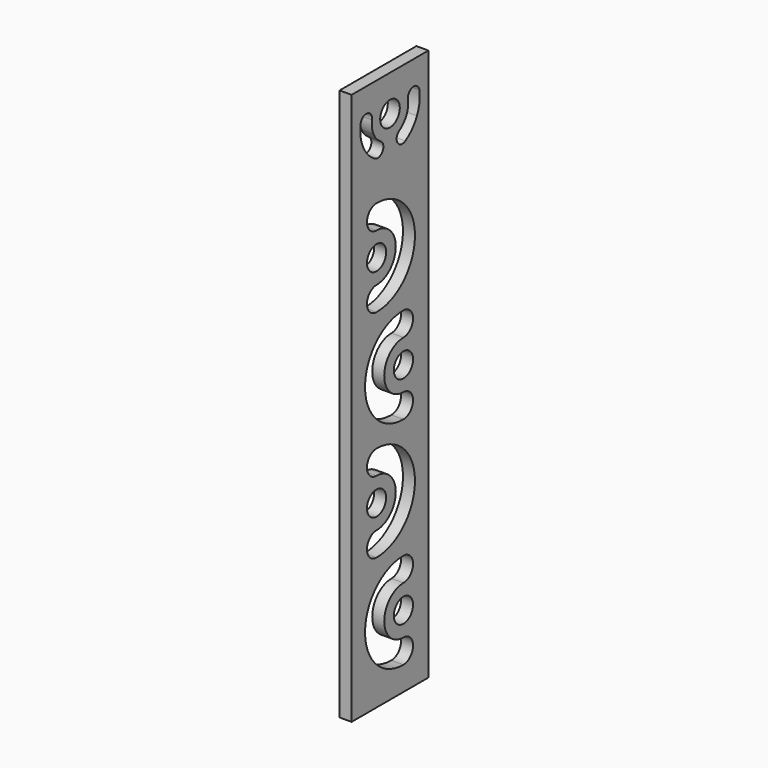
from build123d import *

# Parameters (mm, degrees)
F0_W      = 63.5
F0_H      = 63.5
F0_W_2    = 50.8
F0_H_2    = 50.8
F1_DEPTH  = 165.1
F3_R      = 6.477
F4_DEPTH  = 25.4
F6_DEPTH  = 25.4
F7_R      = 6.35
F8_DEPTH  = 63.501
F9_W      = 93.0855199695
F9_H      = 380.0157606602
F9_W_2    = 50.8
F9_H_2    = 292.1
F10_DEPTH = 38.1
F11_W     = 93.9574092627
F11_H     = 381.9095790386
F12_DEPTH = 91.44


# Not quite as in the source:
# - ends of sketch curves that miss each other by under 0.0002 mm in the source are joined


with BuildPart() as f1:
    # F0 (on Top) → F1 (new body, symmetric)
    with BuildSketch(Plane.XY):
        Rectangle(F0_W, F0_H)
        Rectangle(F0_W_2, F0_H_2, mode=Mode.SUBTRACT)
    extrude(amount=F1_DEPTH, both=True)

    # F3 (on face) → F4 (cut)
    with BuildSketch(Plane.YZ.offset(31.75)):
        with Locations((0, 146.05)):
            Circle(F3_R)
        with BuildLine():
            ThreePointArc((10.1385245046, 129.1766616857), (14.6288058895, 132.8781640138), (17.8406687878, 137.7307595176))
            ThreePointArc((17.8406687878, 137.7307595176), (19.4934269332, 143.3103775076), (19.4426449846, 149.1294124443))
            ThreePointArc((19.4426449846, 149.1294124443), (15.0835370951, 152.2964897102), (11.9164598293, 147.9373818207))
            ThreePointArc((11.9164598293, 147.9373818207), (11.9475842494, 144.3708765369), (10.9346034506, 140.9511106721))
            ThreePointArc((10.9346034506, 140.9511106721), (8.9660423194, 137.9769392343), (6.2139343738, 135.708276517))
            ThreePointArc((6.2139343738, 135.708276517), (4.9104220235, 130.4801740359), (10.1385245046, 129.1766616857))
        make_face()
        with BuildLine():
            ThreePointArc((-10.1385245046, 129.1766616857), (-4.9104220235, 130.4801740359), (-6.2139343738, 135.708276517))
            ThreePointArc((-6.2139343738, 135.708276517), (-8.9660423194, 137.9769392343), (-10.9346034506, 140.9511106721))
            ThreePointArc((-10.9346034506, 140.9511106721), (-11.9475842494, 144.3708765369), (-11.9164598293, 147.9373818207))
            ThreePointArc((-11.9164598293, 147.9373818207), (-15.0835370951, 152.2964897102), (-19.4426449846, 149.1294124443))
            ThreePointArc((-19.4426449846, 149.1294124443), (-19.4934269332, 143.3103775076), (-17.8406687878, 137.7307595176))
            ThreePointArc((-17.8406687878, 137.7307595176), (-14.6288058895, 132.8781640138), (-10.1385245046, 129.1766616857))
        make_face()
    extrude(amount=-F4_DEPTH, mode=Mode.SUBTRACT)

    # F5 (on face) → F6 (cut)
    with BuildSketch(Plane(origin=(-31.75, 0, 0), x_dir=(0, -1, 0), z_dir=(-1, 0, 0))):
        with BuildLine():
            ThreePointArc((-3.1401119103, 140.3850881569), (3.2873259769, 140.4692279278), (6.477, 146.05))
            ThreePointArc((6.477, 146.05), (-3.2873259769, 151.6307720722), (-3.1401119103, 140.3850881569))
        make_face()
        with BuildLine():
            ThreePointArc((-5.7913527214, 132.1654121492), (-6.0549491708, 133.1322727306), (-6.7727903948, 133.8315626913))
            ThreePointArc((-6.7727903948, 133.8315626913), (-9.3377562721, 131.1985515677), (-5.7913527214, 132.1654121492))
        make_face()
        with BuildLine():
            ThreePointArc((3.1226517792, 134.3961049058), (0.4285749428, 129.7298269458), (5.0948529028, 127.0357501095))
            ThreePointArc((5.0948529028, 127.0357501095), (17.8406687878, 137.7307595176), (17.8406687878, 154.3692404824))
            ThreePointArc((17.8406687878, 154.3692404824), (12.777460542, 156.2120975737), (10.9346034506, 151.1488893279))
            ThreePointArc((10.9346034506, 151.1488893279), (10.9346034506, 140.9511106721), (3.1226517792, 134.3961049058))
        make_face()
    extrude(amount=-F6_DEPTH, mode=Mode.SUBTRACT)

    # F7 (on face) → F8 (cut, through all)
    with BuildSketch(Plane.YZ.offset(31.75)):
        with BuildLine():
            ThreePointArc((-8.89, 107.949999693), (-15.239999693, 101.6), (-8.89, 95.250000307))
            ThreePointArc((-8.89, 95.250000307), (3.81, 82.55), (-8.89, 69.85))
            ThreePointArc((-8.89, 69.85), (-15.239999693, 63.5), (-8.89, 57.150000307))
            ThreePointArc((-8.89, 57.150000307), (16.509999693, 82.55), (-8.89, 107.949999693))
        make_face()
        with BuildLine():
            ThreePointArc((8.89, 3.07e-07), (15.239999693, 6.35), (8.89, 12.699999693))
            ThreePointArc((8.89, 12.699999693), (-3.81, 25.4), (8.89, 38.1))
            ThreePointArc((8.89, 38.1), (15.24, 44.45), (8.89, 50.8))
            ThreePointArc((8.89, 50.8), (-16.509999693, 25.4), (8.89, 3.07e-07))
        make_face()
        with BuildLine():
            ThreePointArc((-8.89, -6.350000307), (-15.239999693, -12.7), (-8.89, -19.049999693))
            ThreePointArc((-8.89, -19.049999693), (3.81, -31.75), (-8.89, -44.45))
            ThreePointArc((-8.89, -44.45), (-15.239999693, -50.8), (-8.89, -57.149999693))
            ThreePointArc((-8.89, -57.149999693), (16.509999693, -31.75), (-8.89, -6.350000307))
        make_face()
        with BuildLine():
            ThreePointArc((8.89, -114.299999693), (15.239999693, -107.95), (8.89, -101.600000307))
            ThreePointArc((8.89, -101.600000307), (-3.81, -88.9), (8.89, -76.2))
            ThreePointArc((8.89, -76.2), (15.24, -69.85), (8.89, -63.5))
            ThreePointArc((8.89, -63.5), (-16.509999693, -88.9), (8.89, -114.299999693))
        make_face()
        with Locations((-8.89, 82.55)):
            Circle(F7_R)
        with Locations((8.89, 25.4)):
            Circle(F7_R)
        with Locations((8.89, -88.9)):
            Circle(F7_R)
        with Locations((-8.89, -31.75)):
            Circle(F7_R)
    extrude(amount=-F8_DEPTH, mode=Mode.SUBTRACT)

    # F9 (on face) → F10 (cut, symmetric)
    with BuildSketch(Plane(origin=(25.4, 0, 0), x_dir=(0, -1, 0), z_dir=(-1, 0, 0))):
        Rectangle(F9_W, F9_H)
        with Locations((0, 19.05)):
            Rectangle(F9_W_2, F9_H_2, mode=Mode.SUBTRACT)
    extrude(amount=F10_DEPTH, both=True, mode=Mode.SUBTRACT)

    # F11 (on face) → F12 (cut)
    with BuildSketch(Plane(origin=(25.4, 0, 0), x_dir=(0, -1, 0), z_dir=(-1, 0, 0))):
        Rectangle(F11_W, F11_H)
    extrude(amount=F12_DEPTH, mode=Mode.SUBTRACT)


solid = f1.part
